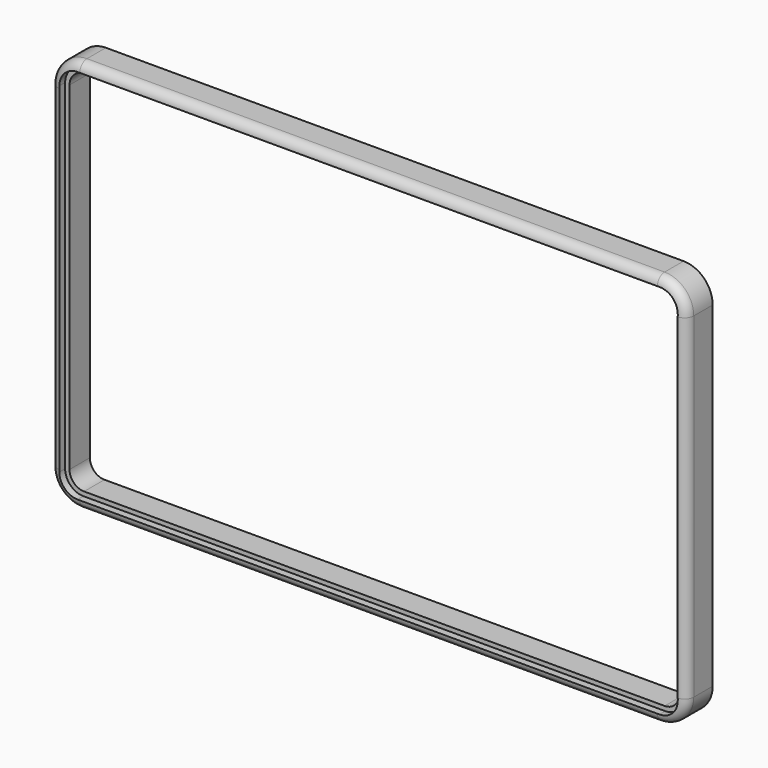
from build123d import *

# Parameters (mm, degrees)
F0_W         = 174.7
F0_H         = 108.2
F0_W_2       = 169.9
F0_H_2       = 103.4
F1_DEPTH     = 2
F0_W_3       = 167.5
F0_H_3       = 101
F2_DEPTH     = 7
F3_R         = 4
F4_R         = 5
F5_R         = 8
F6_T1_DEPTH  = 158.7
F6_T3_DEPTH  = 92.2
F6_T6_ANGLE  = 90
F6_T8_ANGLE  = 90
F6_T10_ANGLE = 90
F6_T12_ANGLE = 90


# Not quite as in the source:
# - a fillet or chamfer that OpenCascade refuses, or shapes differently, is made with other operations: its cross-section is extruded or revolved along the edge and cut away or added


with BuildPart() as f1:
    # F0 (on Front) → F1 (new body)
    with BuildSketch(Plane.XZ):
        Rectangle(F0_W, F0_H)
        Rectangle(F0_W_2, F0_H_2, mode=Mode.SUBTRACT)
    extrude(amount=F1_DEPTH)

    # F0 (on Front) → F2 (join)
    with BuildSketch(Plane.XZ):
        Rectangle(F0_W, F0_H)
        Rectangle(F0_W_2, F0_H_2, mode=Mode.SUBTRACT)
        Rectangle(F0_W_2, F0_H_2)
        Rectangle(F0_W_3, F0_H_3, mode=Mode.SUBTRACT)
    extrude(amount=-F2_DEPTH)

    # F3
    f3_edges = [f1.edges().sort_by_distance(p)[0] for p in [
        (83.75, 3.5, 50.5),
        (-83.75, 3.5, 50.5),
        (-83.75, 3.5, -50.5),
        (83.75, 3.5, -50.5),
    ]]
    fillet(f3_edges, radius=F3_R)

    # F4
    f4_edges = [f1.edges().sort_by_distance(p)[0] for p in [
        (84.95, -1, 51.7),
        (84.95, -1, -51.7),
        (-84.95, -1, -51.7),
        (-84.95, -1, 51.7),
    ]]
    fillet(f4_edges, radius=F4_R)

    # F5
    f5_edges = [f1.edges().sort_by_distance(p)[0] for p in [
        (87.35, 2.5, -54.1),
        (-87.35, 2.5, -54.1),
        (-87.35, 2.5, 54.1),
        (87.35, 2.5, 54.1),
    ]]
    fillet(f5_edges, radius=F5_R)

    # F6: fillet of radius 2.5 on 1 edges, made by hand

    # F6_s2 → F6_t1 (cut)
    with BuildSketch(Plane.YZ.offset(-79.35)):
        with BuildLine():
            ThreePointArc((-2, 51.6), (-1.267766953, 53.367766953), (0.5, 54.1))
            Line((0.5, 54.1), (-2, 54.1))
            Line((-2, 54.1), (-2, 51.6))
        make_face()
        with BuildLine():
            ThreePointArc((-2, -51.6), (-1.267766953, -53.367766953), (0.5, -54.1))
            Line((0.5, -54.1), (-2, -54.1))
            Line((-2, -54.1), (-2, -51.6))
        make_face()
    extrude(amount=F6_T1_DEPTH, mode=Mode.SUBTRACT)

    # F6_s4 → F6_t3 (cut)
    with BuildSketch(Plane.XY.offset(-46.1)):
        with BuildLine():
            ThreePointArc((-84.85, -2), (-86.617766953, -1.267766953), (-87.35, 0.5))
            Line((-87.35, 0.5), (-87.35, -2))
            Line((-87.35, -2), (-84.85, -2))
        make_face()
        with BuildLine():
            ThreePointArc((84.85, -2), (86.617766953, -1.267766953), (87.35, 0.5))
            Line((87.35, 0.5), (87.35, -2))
            Line((87.35, -2), (84.85, -2))
        make_face()
    extrude(amount=F6_T3_DEPTH, mode=Mode.SUBTRACT)

    # F6_s5 → F6_t6 (revolve, cut)
    with BuildSketch(Plane.YZ.offset(-79.35)):
        with BuildLine():
            ThreePointArc((-2, 51.6), (-1.267766953, 53.367766953), (0.5, 54.1))
            Line((0.5, 54.1), (-2, 54.1))
            Line((-2, 54.1), (-2, 51.6))
        make_face()
    revolve(axis=Axis((-79.35, -2, 46.1), (0, -1, 0)), revolution_arc=F6_T6_ANGLE, mode=Mode.SUBTRACT)

    # F6_s7 → F6_t8 (revolve, cut)
    with BuildSketch(Plane.XY.offset(-46.1)):
        with BuildLine():
            ThreePointArc((-84.85, -2), (-86.617766953, -1.267766953), (-87.35, 0.5))
            Line((-87.35, 0.5), (-87.35, -2))
            Line((-87.35, -2), (-84.85, -2))
        make_face()
    revolve(axis=Axis((-79.35, -2, -46.1), (0, -1, 0)), revolution_arc=F6_T8_ANGLE, mode=Mode.SUBTRACT)

    # F6_s9 → F6_t10 (revolve, cut)
    with BuildSketch(Plane.XY.offset(-46.1)):
        with BuildLine():
            ThreePointArc((84.85, -2), (86.617766953, -1.267766953), (87.35, 0.5))
            Line((87.35, 0.5), (87.35, -2))
            Line((87.35, -2), (84.85, -2))
        make_face()
    revolve(axis=Axis((79.35, -2, -46.1), (0, 1, 0)), revolution_arc=F6_T10_ANGLE, mode=Mode.SUBTRACT)

    # F6_s11 → F6_t12 (revolve, cut)
    with BuildSketch(Plane.XY.offset(46.1)):
        with BuildLine():
            ThreePointArc((84.85, -2), (86.617766953, -1.267766953), (87.35, 0.5))
            Line((87.35, 0.5), (87.35, -2))
            Line((87.35, -2), (84.85, -2))
        make_face()
    revolve(axis=Axis((79.35, -2, 46.1), (0, -1, 0)), revolution_arc=F6_T12_ANGLE, mode=Mode.SUBTRACT)


solid = f1.part
